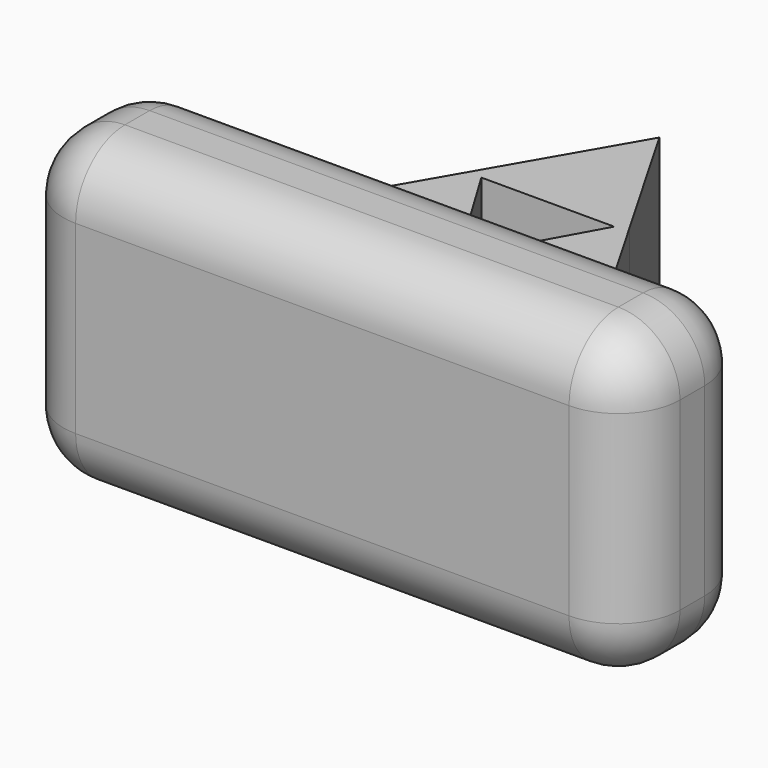
from build123d import *

# Parameters (mm, degrees)
F1_DEPTH = 12.7
F2_DEPTH = 6.35
F4_DEPTH = 19.051
F5_R     = 5.08


# Not quite as in the source:
# - a feature names something its author has since deleted; it is built from what else it names


with BuildPart() as f1:
    # F0 (on Top) → F1 (new body, symmetric)
    with BuildSketch(Plane.XY):
        Polygon((0.2673684239, -2.5617282353), (-12.7, -2.5617282353), (-25.4, -2.5617282353), (-25.4, -15.2617282353), (25.4, -15.2617282353), (25.4, -2.5617282353), (12.7, -2.5617282353), align=None)
    extrude(amount=F1_DEPTH, both=True)

    # F0 (on Top) → F2 (join, symmetric)
    with BuildSketch(Plane.XY):
        Polygon((6.35, 8.4367943928), (0.2673684239, -2.5617282353), (12.7, -2.5617282353), align=None)
        Polygon((-6.35, 8.4367943928), (-12.7, -2.5617282353), (0.2673684239, -2.5617282353), align=None)
        Polygon((0, 19.4353170208), (-6.35, 8.4367943928), (6.35, 8.4367943928), align=None)
        Polygon((-6.35, 8.4367943928), (0.2673684239, -2.5617282353), (6.35, 8.4367943928), align=None)
    extrude(amount=F2_DEPTH, both=True)

    # F3 (on face) → F4 (cut, through all)
    with BuildSketch(Plane.XY.offset(6.35)):
        Polygon((5.4885434949, 7.9287943928), (-5.4514978916, 7.9287943928), (0.2488394649, -1.5455593664), align=None)
    extrude(amount=-F4_DEPTH, mode=Mode.SUBTRACT)

    # F5
    f5_edges = [f1.edges().sort_by_distance(p)[0] for p in [
        (-25.4, -8.911728, 12.7),
        (-25.4, -8.911728, -12.7),
        (25.4, -8.911728, -12.7),
        (25.4, -8.911728, 12.7),
        (-25.4, -15.261728, 0),
        (0, -15.261728, -12.7),
        (25.4, -15.261728, 0),
        (0, -15.261728, 12.7),
        (0, -2.561728, 12.7),
        (0, -2.561728, -12.7),
        (25.4, -2.561728, 0),
        (-25.4, -2.561728, 0),
    ]]
    fillet(f5_edges, radius=F5_R)


solid = f1.part
